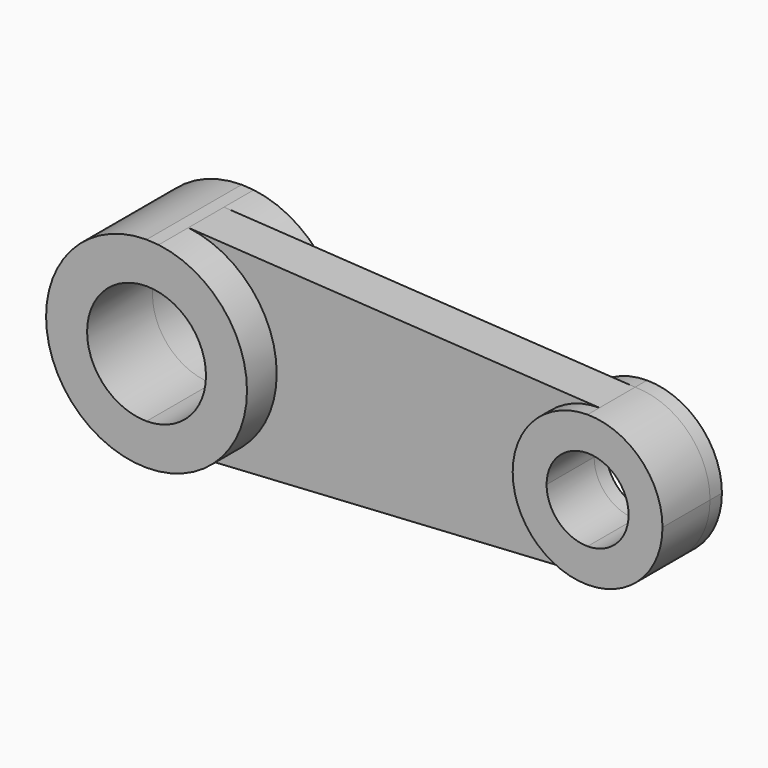
from build123d import *

# Parameters (mm, degrees)
F1_DEPTH = 19.05
F2_DEPTH = 34.925
F3_DEPTH = 25.4
F4_DEPTH = 6.35
F5_DEPTH = 15.875


with BuildPart() as f1:
    # F0 (on Front) → F1 (new body)
    with BuildSketch(Plane.XZ):
        with BuildLine():
            Line((0, -25.4), (0, -42.926))
            Line((0, -42.926), (5.16603969, -42.61400603))
            ThreePointArc((5.16603969, -42.61400603), (32.1278609289, -28.4682635251), (42.926, 0))
            Line((42.926, 0), (25.4, 0))
            ThreePointArc((25.4, 0), (17.9605122421, -17.9605122421), (0, -25.4))
        make_face()
        with BuildLine():
            Line((180.848, 32.004), (5.16603969, 42.61400603))
            ThreePointArc((5.16603969, 42.61400603), (32.1278609289, 28.4682635251), (42.926, 0))
            Line((42.926, 0), (148.844, 0))
            ThreePointArc((148.844, 0), (158.2177545749, 22.6302454251), (180.848, 32.004))
        make_face()
        with BuildLine():
            ThreePointArc((42.926, 0), (32.1278609289, -28.4682635251), (5.16603969, -42.61400603))
            Line((5.16603969, -42.61400603), (180.848, -32.004))
            ThreePointArc((180.848, -32.004), (158.2177545749, -22.6302454251), (148.844, 0))
            Line((148.844, 0), (42.926, 0))
        make_face()
    extrude(amount=F1_DEPTH)

    # F0 (on Front) → F2 (join)
    with BuildSketch(Plane.XZ):
        with BuildLine():
            Line((0, 25.4), (0, 42.926))
            ThreePointArc((0, 42.926), (-42.926, 0), (0, -42.926))
            Line((0, -42.926), (0, -25.4))
            ThreePointArc((0, -25.4), (-25.4, 0), (0, 25.4))
        make_face()
        with BuildLine():
            Line((5.16603969, 42.61400603), (0, 42.926))
            Line((0, 42.926), (0, 25.4))
            ThreePointArc((0, 25.4), (17.9605122421, 17.9605122421), (25.4, 0))
            Line((25.4, 0), (42.926, 0))
            ThreePointArc((42.926, 0), (32.1278609289, 28.4682635251), (5.16603969, 42.61400603))
        make_face()
        with BuildLine():
            Line((0, -25.4), (0, -42.926))
            Line((0, -42.926), (5.16603969, -42.61400603))
            ThreePointArc((5.16603969, -42.61400603), (32.1278609289, -28.4682635251), (42.926, 0))
            Line((42.926, 0), (25.4, 0))
            ThreePointArc((25.4, 0), (17.9605122421, -17.9605122421), (0, -25.4))
        make_face()
    extrude(amount=F2_DEPTH)

    # F0 (on Front) → F3 (join)
    with BuildSketch(Plane.XZ):
        with BuildLine():
            Line((180.848, 17.526), (180.848, 32.004))
            ThreePointArc((180.848, 32.004), (158.2177545749, 22.6302454251), (148.844, 0))
            Line((148.844, 0), (163.322, 0))
            ThreePointArc((163.322, 0), (168.4552465529, 12.3927534471), (180.848, 17.526))
        make_face()
        with BuildLine():
            ThreePointArc((148.844, 0), (158.2177545749, -22.6302454251), (180.848, -32.004))
            Line((180.848, -32.004), (180.848, -17.526))
            ThreePointArc((180.848, -17.526), (168.4552465529, -12.3927534471), (163.322, 0))
            Line((163.322, 0), (148.844, 0))
        make_face()
        with BuildLine():
            ThreePointArc((212.852, 0), (203.4782454251, 22.6302454251), (180.848, 32.004))
            Line((180.848, 32.004), (180.848, 17.526))
            ThreePointArc((180.848, 17.526), (193.2407534471, 12.3927534471), (198.374, 0))
            ThreePointArc((198.374, 0), (193.2407534471, -12.3927534471), (180.848, -17.526))
            Line((180.848, -17.526), (180.848, -32.004))
            ThreePointArc((180.848, -32.004), (203.4782454251, -22.6302454251), (212.852, 0))
        make_face()
    extrude(amount=F3_DEPTH)

    # F0 (on Front) → F4 (join)
    with BuildSketch(Plane.XZ):
        with BuildLine():
            ThreePointArc((212.852, 0), (203.4782454251, 22.6302454251), (180.848, 32.004))
            Line((180.848, 32.004), (180.848, 17.526))
            ThreePointArc((180.848, 17.526), (193.2407534471, 12.3927534471), (198.374, 0))
            ThreePointArc((198.374, 0), (193.2407534471, -12.3927534471), (180.848, -17.526))
            Line((180.848, -17.526), (180.848, -32.004))
            ThreePointArc((180.848, -32.004), (203.4782454251, -22.6302454251), (212.852, 0))
        make_face()
        with BuildLine():
            ThreePointArc((148.844, 0), (158.2177545749, -22.6302454251), (180.848, -32.004))
            Line((180.848, -32.004), (180.848, -17.526))
            ThreePointArc((180.848, -17.526), (168.4552465529, -12.3927534471), (163.322, 0))
            Line((163.322, 0), (148.844, 0))
        make_face()
        with BuildLine():
            Line((180.848, 17.526), (180.848, 32.004))
            ThreePointArc((180.848, 32.004), (158.2177545749, 22.6302454251), (148.844, 0))
            Line((148.844, 0), (163.322, 0))
            ThreePointArc((163.322, 0), (168.4552465529, 12.3927534471), (180.848, 17.526))
        make_face()
    extrude(amount=-F4_DEPTH)

    # F0 (on Front) → F5 (join)
    with BuildSketch(Plane.XZ):
        with BuildLine():
            Line((0, 25.4), (0, 42.926))
            ThreePointArc((0, 42.926), (-42.926, 0), (0, -42.926))
            Line((0, -42.926), (0, -25.4))
            ThreePointArc((0, -25.4), (-25.4, 0), (0, 25.4))
        make_face()
        with BuildLine():
            Line((5.16603969, 42.61400603), (0, 42.926))
            Line((0, 42.926), (0, 25.4))
            ThreePointArc((0, 25.4), (17.9605122421, 17.9605122421), (25.4, 0))
            Line((25.4, 0), (42.926, 0))
            ThreePointArc((42.926, 0), (32.1278609289, 28.4682635251), (5.16603969, 42.61400603))
        make_face()
        with BuildLine():
            Line((0, -25.4), (0, -42.926))
            Line((0, -42.926), (5.16603969, -42.61400603))
            ThreePointArc((5.16603969, -42.61400603), (32.1278609289, -28.4682635251), (42.926, 0))
            Line((42.926, 0), (25.4, 0))
            ThreePointArc((25.4, 0), (17.9605122421, -17.9605122421), (0, -25.4))
        make_face()
    extrude(amount=-F5_DEPTH)


solid = f1.part
